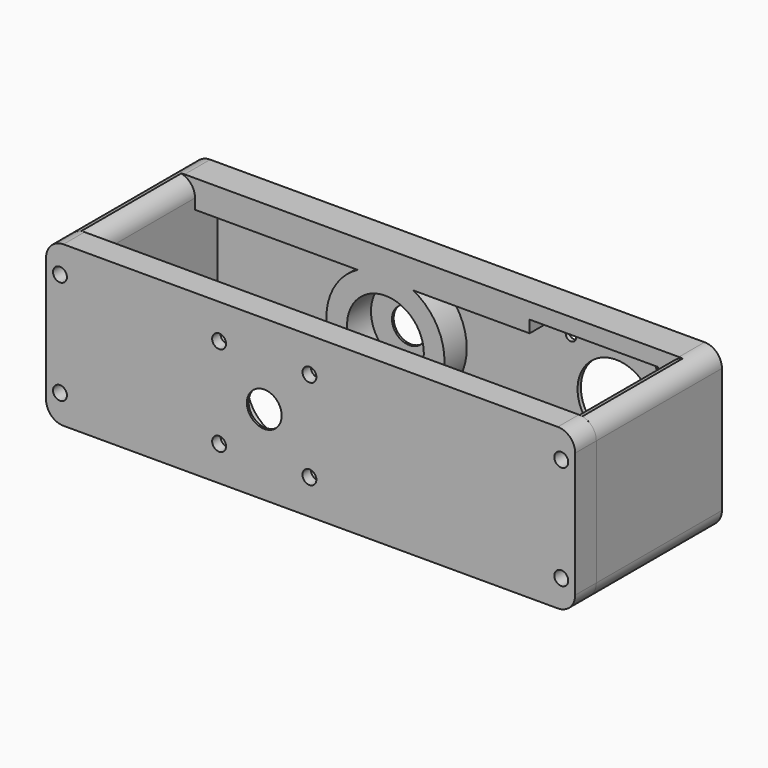
from build123d import *

# Parameters (mm, degrees)
F0_W       = 152.3125
F0_H       = 46
F0_R       = 1.5
F0_R_2     = 11.05
F0_R_3     = 11.1
F1_DEPTH   = 1.2
F2_W       = 152.3125
F2_H       = 46
F2_R       = 11.05
F3_DEPTH   = 8
F4_W       = 8
F4_H       = 46
F5_DEPTH   = 36
F6_W       = 152.3125
F6_H       = 46
F7_DEPTH   = 7.6
F0_R_4     = 5
F8_DEPTH   = 0.6
F9_R       = 11.05
F9_R_2     = 5
F9_R_3     = 2
F10_DEPTH  = 52.801
F11_DEPTH  = 0.6
F14_DEPTH  = 3
F15_R      = 2
F16_DEPTH  = 15
F19_DEPTH  = 3
F20_R      = 2
F21_DEPTH  = 52.801
F22_F1_R   = 5
F22_F2_R   = 5
F22_F3_R   = 5
F22_F4_R   = 5
F22_F5_R   = 5
F22_F6_R   = 5
F22_F7_R   = 5
F22_F8_R   = 5
F22_2_F1_R = 5
F22_2_F2_R = 5
F22_2_F3_R = 5
F22_2_F4_R = 5


with BuildPart() as f1:
    # F0 (on Front) → F1 (new body)
    with BuildSketch(Plane.XZ):
        with Locations((13.34375, 0)):
            Rectangle(F0_W, F0_H)
        with Locations((47, -13)):
            Circle(F0_R, mode=Mode.SUBTRACT)
        with Locations((73, -13)):
            Circle(F0_R, mode=Mode.SUBTRACT)
        Circle(F0_R_2, mode=Mode.SUBTRACT)
        with Locations((60, 0)):
            Circle(F0_R_3, mode=Mode.SUBTRACT)
        with Locations((47, 13)):
            Circle(F0_R, mode=Mode.SUBTRACT)
        with Locations((73, 13)):
            Circle(F0_R, mode=Mode.SUBTRACT)
    extrude(amount=F1_DEPTH)

    # F2 (on face) → F3 (join)
    with BuildSketch(Plane.XZ.offset(1.2)):
        with Locations((13.34375, 0)):
            Rectangle(F2_W, F2_H)
        with BuildLine():
            Line((-8, -15), (-54.8125, -15))
            Line((-54.8125, -15), (-54.8125, 15))
            Line((-54.8125, 15), (-8, 15))
            ThreePointArc((-8, 15), (-17, 0), (-8, -15))
        make_face(mode=Mode.SUBTRACT)
        Circle(F2_R, mode=Mode.SUBTRACT)
        with BuildLine():
            Line((78.5, 15), (81.5, 15))
            Line((81.5, 15), (81.5, -15))
            Line((81.5, -15), (78.5, -15))
            Line((78.5, -15), (78.5, -18.5))
            Line((78.5, -18.5), (41.5, -18.5))
            Line((41.5, -18.5), (41.5, -15))
            Line((41.5, -15), (8, -15))
            ThreePointArc((8, -15), (17, 0), (8, 15))
            Line((8, 15), (41.5, 15))
            Line((41.5, 15), (41.5, 18.5))
            Line((41.5, 18.5), (78.5, 18.5))
            Line((78.5, 18.5), (78.5, 15))
        make_face(mode=Mode.SUBTRACT)
    extrude(amount=F3_DEPTH)

    # F4 (on face) → F5 (join)
    with BuildSketch(Plane.XZ.offset(9.2)):
        with Locations((85.5, 0)):
            Rectangle(F4_W, F4_H)
        with Locations((-58.8125, 0)):
            Rectangle(F4_W, F4_H)
    extrude(amount=F5_DEPTH)

    # F0 (on Front) → F8 (join)
    with BuildSketch(Plane.XZ):
        Circle(F0_R_2)
        Circle(F0_R_4, mode=Mode.SUBTRACT)
    extrude(amount=F8_DEPTH)

    # F15 (on face) → F16 (cut)
    with BuildSketch(Plane.XZ.offset(45.2)):
        with Locations((85.5, 15)):
            Circle(F15_R)
        with Locations((85.5, -15)):
            Circle(F15_R)
        with Locations((-58.8125, 15)):
            Circle(F15_R)
        with Locations((-58.8125, -15)):
            Circle(F15_R)
    extrude(amount=-F16_DEPTH, mode=Mode.SUBTRACT)

    # F18 (on offset) → F19 (cut)
    with BuildSketch(Plane.XZ.offset(40.2)):
        Polygon((-55.1125, 12.863804004), (-55.1125, 17.136195996), (-58.8125, 19.272391992), (-62.5125, 17.136195996), (-62.5125, 12.863804004), (-58.8125, 10.727608008), align=None)
        Polygon((-55.1125, -17.136195996), (-55.1125, -12.863804004), (-58.8125, -10.727608008), (-62.5125, -12.863804004), (-62.5125, -17.136195996), (-58.8125, -19.272391992), align=None)
        Polygon((81.8, 17.136195996), (81.8, 12.863804004), (85.5, 10.727608008), (89.2, 12.863804004), (89.2, 17.136195996), (85.5, 19.272391992), align=None)
        Polygon((81.8, -12.863804004), (81.8, -17.136195996), (85.5, -19.272391992), (89.2, -17.136195996), (89.2, -12.863804004), (85.5, -10.727608008), align=None)
    extrude(amount=-F19_DEPTH, mode=Mode.SUBTRACT)

    # F22: fillet of radius 5 on 8 edges, made by hand

    # F22_f1
    f22_f1_edges = [f1.edges().sort_by_distance(p)[0] for p in [
        (81.5, -27.2, 23),
    ]]
    fillet(f22_f1_edges, radius=F22_F1_R)

    # F22_f2
    f22_f2_edges = [f1.edges().sort_by_distance(p)[0] for p in [
        (-54.8125, -27.2, 23),
    ]]
    fillet(f22_f2_edges, radius=F22_F2_R)

    # F22_f3
    f22_f3_edges = [f1.edges().sort_by_distance(p)[0] for p in [
        (81.5, -27.2, -23),
    ]]
    fillet(f22_f3_edges, radius=F22_F3_R)

    # F22_f4
    f22_f4_edges = [f1.edges().sort_by_distance(p)[0] for p in [
        (-54.8125, -27.2, -23),
    ]]
    fillet(f22_f4_edges, radius=F22_F4_R)

    # F22_f5
    f22_f5_edges = [f1.edges().sort_by_distance(p)[0] for p in [
        (89.5, -22.6, 23),
    ]]
    fillet(f22_f5_edges, radius=F22_F5_R)

    # F22_f6
    f22_f6_edges = [f1.edges().sort_by_distance(p)[0] for p in [
        (-62.8125, -22.6, 23),
    ]]
    fillet(f22_f6_edges, radius=F22_F6_R)

    # F22_f7
    f22_f7_edges = [f1.edges().sort_by_distance(p)[0] for p in [
        (89.5, -22.6, -23),
    ]]
    fillet(f22_f7_edges, radius=F22_F7_R)

    # F22_f8
    f22_f8_edges = [f1.edges().sort_by_distance(p)[0] for p in [
        (-62.8125, -22.6, -23),
    ]]
    fillet(f22_f8_edges, radius=F22_F8_R)


with BuildPart() as f7:
    # F6 (on face) → F7 (new body)
    with BuildSketch(Plane.XZ.offset(45.2)):
        with Locations((13.34375, 0)):
            Rectangle(F6_W, F6_H)
    extrude(amount=F7_DEPTH)

    # F9 (on face) → F10 (cut, through all)
    with BuildSketch(Plane.XZ.offset(52.8)):
        Circle(F9_R)
        Circle(F9_R_2, mode=Mode.SUBTRACT)
        with Locations((-13, -13)):
            Circle(F9_R_3)
        with Locations((13, -13)):
            Circle(F9_R_3)
        with Locations((13, 13)):
            Circle(F9_R_3)
        with Locations((-13, 13)):
            Circle(F9_R_3)
        Circle(F9_R_2)
    extrude(amount=-F10_DEPTH, mode=Mode.SUBTRACT)

    # F9 (on face) → F11 (join)
    with BuildSketch(Plane.XZ.offset(52.8)):
        Circle(F9_R)
        Circle(F9_R_2, mode=Mode.SUBTRACT)
    extrude(amount=-F11_DEPTH)

    # F13 (on offset) → F14 (cut)
    with BuildSketch(Plane.XZ.offset(49.8)):
        Polygon((-9.3, -15.136195996), (-9.3, -10.863804004), (-13, -8.727608008), (-16.7, -10.863804004), (-16.7, -15.136195996), (-13, -17.272391992), align=None)
        Polygon((-9.3, 10.863804004), (-9.3, 15.136195996), (-13, 17.272391992), (-16.7, 15.136195996), (-16.7, 10.863804004), (-13, 8.727608008), align=None)
        Polygon((9.3, 15.136195996), (9.3, 10.863804004), (13, 8.727608008), (16.7, 10.863804004), (16.7, 15.136195996), (13, 17.272391992), align=None)
        Polygon((9.3, -10.863804004), (9.3, -15.136195996), (13, -17.272391992), (16.7, -15.136195996), (16.7, -10.863804004), (13, -8.727608008), align=None)
    extrude(amount=-F14_DEPTH, mode=Mode.SUBTRACT)

    # F20 (on face) → F21 (cut, through all)
    with BuildSketch(Plane.XZ.offset(52.8)):
        with Locations((-58.8125, -15)):
            Circle(F20_R)
        with Locations((-58.8125, 15)):
            Circle(F20_R)
        with Locations((85.5, 15)):
            Circle(F20_R)
        with Locations((85.5, -15)):
            Circle(F20_R)
    extrude(amount=-F21_DEPTH, mode=Mode.SUBTRACT)

    # F22#2: fillet of radius 5 on 4 edges, made by hand

    # F22_2_f1
    f22_2_f1_edges = [f7.edges().sort_by_distance(p)[0] for p in [
        (-62.8125, -49, -23),
    ]]
    fillet(f22_2_f1_edges, radius=F22_2_F1_R)

    # F22_2_f2
    f22_2_f2_edges = [f7.edges().sort_by_distance(p)[0] for p in [
        (89.5, -49, -23),
    ]]
    fillet(f22_2_f2_edges, radius=F22_2_F2_R)

    # F22_2_f3
    f22_2_f3_edges = [f7.edges().sort_by_distance(p)[0] for p in [
        (-62.8125, -49, 23),
    ]]
    fillet(f22_2_f3_edges, radius=F22_2_F3_R)

    # F22_2_f4
    f22_2_f4_edges = [f7.edges().sort_by_distance(p)[0] for p in [
        (89.5, -49, 23),
    ]]
    fillet(f22_2_f4_edges, radius=F22_2_F4_R)


solid = Compound([f1.part, f7.part])
